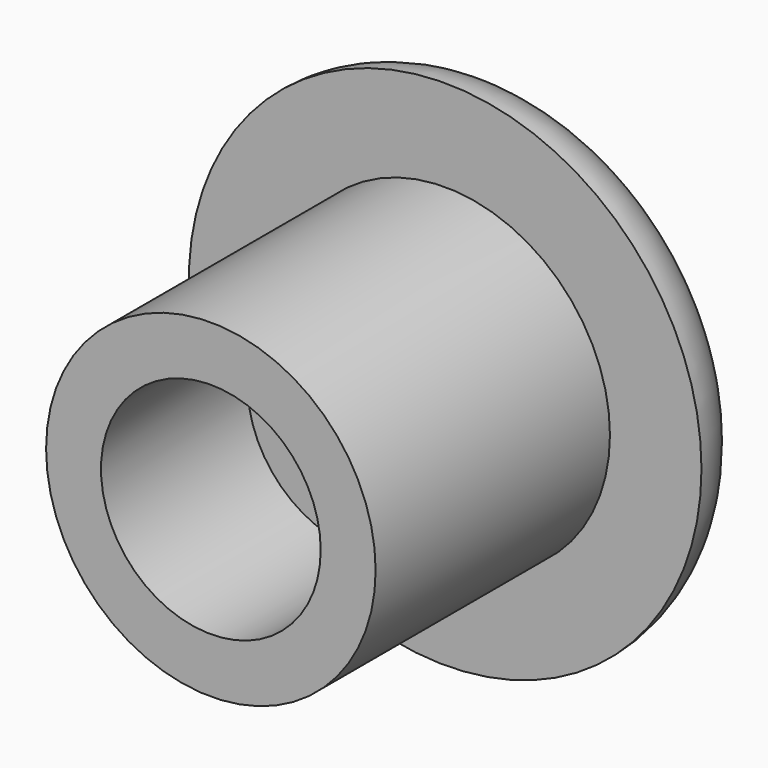
from build123d import *

# Parameters (mm, degrees)
F0_R     = 4.5
F1_DEPTH = 8
F0_R_2   = 7
F2_DEPTH = 2
F3_R     = 1.99999
F4_R     = 3
F5_DEPTH = 5


# Not quite as in the source:
# - a fillet or chamfer is up to 0.001 mm smaller than in the source, because OpenCascade refuses the exact size


with BuildPart() as f1:
    # F0 (on Front) → F1 (new body)
    with BuildSketch(Plane.XZ):
        Circle(F0_R)
    extrude(amount=F1_DEPTH)

    # F0 (on Front) → F2 (join)
    with BuildSketch(Plane.XZ):
        Circle(F0_R_2)
        Circle(F0_R, mode=Mode.SUBTRACT)
        Circle(F0_R)
    extrude(amount=-F2_DEPTH)

    # F3 (radius 2 in the source; OpenCascade refuses exactly that, so slightly less here)
    f3_edges = [f1.edges().sort_by_distance(p)[0] for p in [
        (-7, 2, 0),
    ]]
    fillet(f3_edges, radius=F3_R)

    # F4 (on face) → F5 (cut)
    with BuildSketch(Plane.XZ.offset(8)):
        Circle(F4_R)
    extrude(amount=-F5_DEPTH, mode=Mode.SUBTRACT)


solid = f1.part
